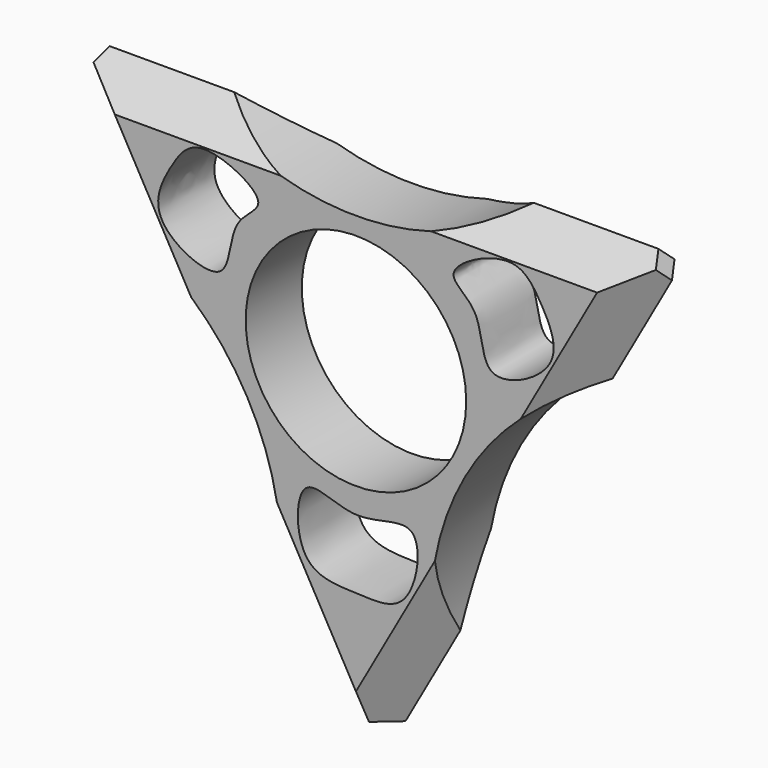
from build123d import *

# Parameters (mm, degrees)
F0_R         = 11
F1_DEPTH     = 7
F2_T1_DEPTH  = 35.2813832436
F2_T3_DEPTH  = 35.5467430765
F2_T5_DEPTH  = 34.4305362998
F2_T7_DEPTH  = 34.4305362998
F2_T9_DEPTH  = 35.2813832436
F2_T11_DEPTH = 35.5467430765


# Not quite as in the source:
# - a fillet or chamfer that OpenCascade refuses, or shapes differently, is made with other operations: its cross-section is extruded or revolved along the edge and cut away or added


with BuildPart() as f1:
    # F0 (on Front) → F1 (new body)
    with BuildSketch(Plane.XZ):
        with BuildLine():
            Line((-8.017778225, -25.1282889185), (-3.9536927291, -32.3677882552))
            Line((-3.9536927291, -32.3677882552), (3.9536927291, -32.3677882552))
            Line((3.9536927291, -32.3677882552), (8.017778225, -25.1282889185))
            ThreePointArc((8.017778225, -25.1282889185), (10.8745416094, -6.6499044579), (25.1621004057, 5.4114989824))
            Line((25.1621004057, 5.4114989824), (29.6426898708, 13.3929315811))
            Line((29.6426898708, 13.3929315811), (26.4639375252, 18.8986921484))
            Line((26.4639375252, 18.8986921484), (17.0454936065, 18.8986921484))
            ThreePointArc((17.0454936065, 18.8986921484), (0, 12.7406410493), (-17.0454936065, 18.8986921484))
            Line((-17.0454936065, 18.8986921484), (-26.4639375252, 18.8986921484))
            Line((-26.4639375252, 18.8986921484), (-29.6426898708, 13.3929315811))
            Line((-29.6426898708, 13.3929315811), (-25.1621004057, 5.4114989824))
            ThreePointArc((-25.1621004057, 5.4114989824), (-12.3306252771, -4.3414248541), (-7.4606163281, -19.7053205246))
            ThreePointArc((-7.4606163281, -19.7053205246), (-7.6002724535, -22.4310780148), (-8.017778225, -25.1282889185))
        make_face()
        Circle(F0_R, mode=Mode.SUBTRACT)
        with BuildLine():
            add(Edge.make_bspline(
                [(-19.3436696139, 6.063790572), (-18.3265059586, 4.2478718705), (-12.0994972205, 1.2345505969), (-12.9508733301, 8.6848868215), (-7.5736250413, 10.7848154742), (-15.8181364049, 15.0617341011), (-18.5131317461, 11.1739776744), (-20.2594400544, 7.6986943169), (-19.3436696139, 6.063790572)],
                knots=[0, 0, 0, 0, 0.1871980652, 0.3557946644, 0.4941971016, 0.6784835343, 0.8314622689, 1, 1, 1, 1], degree=3))
        make_face(mode=Mode.SUBTRACT)
        with BuildLine():
            add(Edge.make_bspline(
                [(-4.9653253518, -12.7779729664), (-3.9673538813, -11.990438984), (-0.0815721197, -14.8647438543), (7.1063785889, -10.9230753891), (5.7028649477, -20.847724526), (0.130602412, -20.2827447937), (-6.1063753916, -20.3844092682), (-6.0569718905, -13.6394292017), (-4.9653253518, -12.7779729664)],
                knots=[0, 0, 0, 0, 0.1595531099, 0.3282047144, 0.5033592864, 0.6613074183, 0.8254703614, 1, 1, 1, 1], degree=3))
        make_face(mode=Mode.SUBTRACT)
        with BuildLine():
            add(Edge.make_bspline(
                [(19.3436696139, 6.063790572), (18.3265059586, 4.2478718705), (12.0994972205, 1.2345505969), (12.9508733301, 8.6848868215), (7.5736250413, 10.7848154742), (15.8181364049, 15.0617341011), (18.5131317461, 11.1739776744), (20.2594400544, 7.6986943169), (19.3436696139, 6.063790572)],
                knots=[0, 0, 0, 0, 0.1871980652, 0.3557946644, 0.4941971016, 0.6784835343, 0.8314622689, 1, 1, 1, 1], degree=3))
        make_face(mode=Mode.SUBTRACT)
    extrude(amount=F1_DEPTH)

    # F2: chamfer of 5.08 on 12 edges, made by hand

    # F2_s2 → F2_t1 (cut)
    with BuildSketch(Plane(origin=(-19.2151547034, 0, 34.2286351679), x_dir=(0, 1, 0), z_dir=(0.4895169129, 0, -0.8719938027))):
        Polygon((-7, -14.2121753414), (-1.92, -19.2921753414), (-7, -19.2921753414), align=None)
        Polygon((-5.08, -19.2921753414), (0, -14.2121753414), (0, -19.2921753414), align=None)
    extrude(amount=F2_T1_DEPTH, mode=Mode.SUBTRACT)

    # F2_s4 → F2_t3 (cut)
    with BuildSketch(Plane.YZ.offset(-39.5280871041)):
        Polygon((-7, 13.8186921484), (-1.92, 18.8986921484), (-7, 18.8986921484), align=None)
        Polygon((-5.08, 18.8986921484), (0, 13.8186921484), (0, 18.8986921484), align=None)
    extrude(amount=F2_T3_DEPTH, mode=Mode.SUBTRACT)

    # F2_s6 → F2_t5 (cut)
    with BuildSketch(Plane(origin=(-19.2640867811, 0, -34.3157996098), x_dir=(0, 1, 0), z_dir=(0.4895169129, 0, 0.8719938027))):
        Polygon((-7, -14.2121753414), (-1.92, -19.2921753414), (-7, -19.2921753414), align=None)
        Polygon((-5.08, -19.2921753414), (0, -14.2121753414), (0, -19.2921753414), align=None)
    extrude(amount=F2_T5_DEPTH, mode=Mode.SUBTRACT)

    # F2_s8 → F2_t7 (cut)
    with BuildSketch(Plane(origin=(2.4097569425, 0, -4.2925853318), x_dir=(0, 1, 0), z_dir=(0.4895169129, 0, -0.8719938027))):
        Polygon((-1.92, -19.2921753414), (-7, -14.2121753414), (-7, -19.2921753414), align=None)
        Polygon((-5.08, -19.2921753414), (0, -14.2121753414), (0, -19.2921753414), align=None)
    extrude(amount=F2_T7_DEPTH, mode=Mode.SUBTRACT)

    # F2_s10 → F2_t9 (cut)
    with BuildSketch(Plane(origin=(1.9443208955, 0, 3.4634876278), x_dir=(0, 1, 0), z_dir=(0.4895169129, 0, 0.8719938027))):
        Polygon((-7, -14.2121753414), (-1.92, -19.2921753414), (-7, -19.2921753414), align=None)
        Polygon((-5.08, -19.2921753414), (0, -14.2121753414), (0, -19.2921753414), align=None)
    extrude(amount=F2_T9_DEPTH, mode=Mode.SUBTRACT)

    # F2_s12 → F2_t11 (cut)
    with BuildSketch(Plane.YZ.offset(3.9813440276)):
        Polygon((-7, 13.8186921484), (-1.92, 18.8986921484), (-7, 18.8986921484), align=None)
        Polygon((-5.08, 18.8986921484), (0, 13.8186921484), (0, 18.8986921484), align=None)
    extrude(amount=F2_T11_DEPTH, mode=Mode.SUBTRACT)


solid = f1.part
